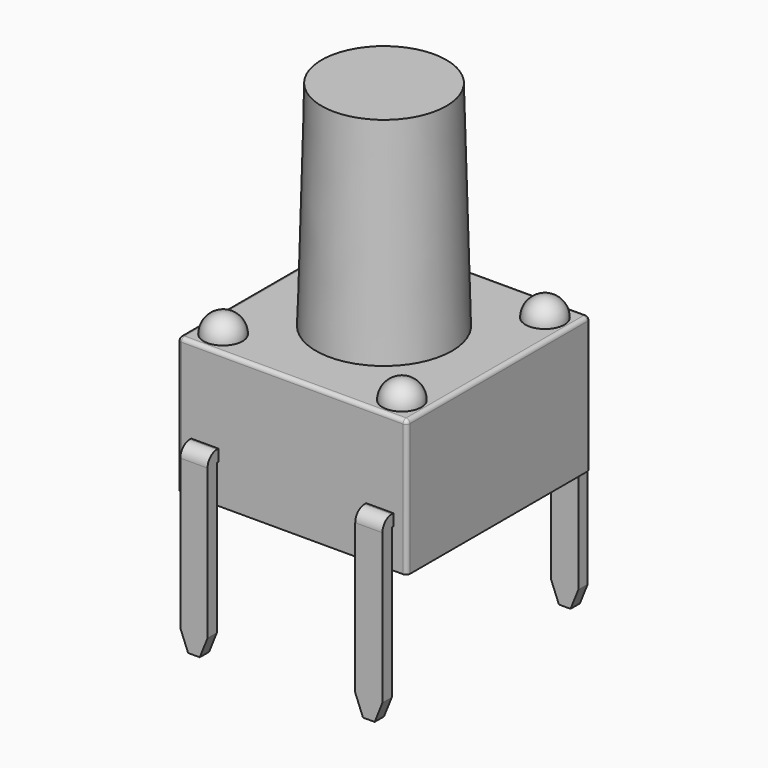
from build123d import *

# Parameters (mm, degrees)
F0_W        = 5.9
F0_H        = 5.9
F1_DEPTH    = 3.5
F2_R        = 1.75
F3_DEPTH    = 5.5
F3_TAPER    = 1.5
F4_R        = 0.1
F5_R        = 0.5
F6_DEPTH    = 0.5
F7_R        = 0.49999
F8_W        = 0.7
F8_H        = 0.3
F11_SIZE2   = 0.5
F11_SIZE    = 0.2
F11_2_SIZE2 = 0.5
F11_2_SIZE  = 0.2


# Not quite as in the source:
# - a fillet or chamfer is up to 0.001 mm smaller than in the source, because OpenCascade refuses the exact size


with BuildPart() as f1:
    # F0 (on Top) → F1 (new body)
    with BuildSketch(Plane.XY):
        Rectangle(F0_W, F0_H)
    extrude(amount=F1_DEPTH)

    # F2 (on face) → F3 (join)
    with BuildSketch(Plane.XY.offset(3.5)):
        Circle(F2_R)
    extrude(amount=F3_DEPTH, taper=F3_TAPER)

    # F4
    f4_edges = [f1.edges().sort_by_distance(p)[0] for p in [
        (2.95, -2.95, 1.75),
        (-2.95, -2.95, 1.75),
        (-2.95, 2.95, 1.75),
        (2.95, 2.95, 1.75),
        (2.95, 0, 3.5),
        (0, -2.95, 3.5),
        (-2.95, 0, 3.5),
        (0, 2.95, 3.5),
    ]]
    fillet(f4_edges, radius=F4_R)

    # F5 (on face) → F6 (join)
    with BuildSketch(Plane.XY.offset(3.5)):
        with Locations((2.3, -2.3)):
            Circle(F5_R)
        with Locations((2.3, 2.3)):
            Circle(F5_R)
        with Locations((-2.3, 2.3)):
            Circle(F5_R)
        with Locations((-2.3, -2.3)):
            Circle(F5_R)
    extrude(amount=F6_DEPTH)

    # F7 (radius 0.5 in the source; OpenCascade refuses exactly that, so slightly less here)
    f7_edges = [f1.edges().sort_by_distance(p)[0] for p in [
        (1.8, -2.3, 4),
        (1.8, 2.3, 4),
        (-2.8, 2.3, 4),
        (-2.8, -2.3, 4),
    ]]
    fillet(f7_edges, radius=F7_R)

    # F10: sweep along a path in F9
    with BuildLine(Plane.YZ) as f10_path:
        Line((-2.95, 1.15), (-3, 1.15))
        ThreePointArc((-3, 1.15), (-3.1060660172, 1.1060660172), (-3.15, 1))
        Line((-3.15, 1), (-3.15, -3.35))
    # F8 (on face) → F10 (sweep)
    with BuildSketch(Plane.XZ.offset(2.95)):
        with Locations((-2.25, 1.15)):
            Rectangle(F8_W, F8_H)
        with Locations((2.25, 1.15)):
            Rectangle(F8_W, F8_H)
    sweep(path=f10_path.line)

    # F11
    f11_edges = [f1.edges().sort_by_distance(p)[0] for p in [
        (-2.6, -3.15, -3.35),
        (-1.9, -3.15, -3.35),
    ]]
    f11_side = f1.faces().sort_by_distance((-2.25, -3.15, -3.35))[0]
    chamfer(f11_edges, length=F11_SIZE, length2=F11_SIZE2, reference=f11_side)

    # F11#2
    f11_2_edges = [f1.edges().sort_by_distance(p)[0] for p in [
        (1.9, -3.15, -3.35),
        (2.6, -3.15, -3.35),
    ]]
    f11_2_side = f1.faces().sort_by_distance((2.25, -3.15, -3.35))[0]
    chamfer(f11_2_edges, length=F11_2_SIZE, length2=F11_2_SIZE2, reference=f11_2_side)

    # F12: F1 across plane


with BuildPart() as f1_1:
    add(f1.part)
    add(f1.part.mirror(Plane.XZ))


solid = f1_1.part
